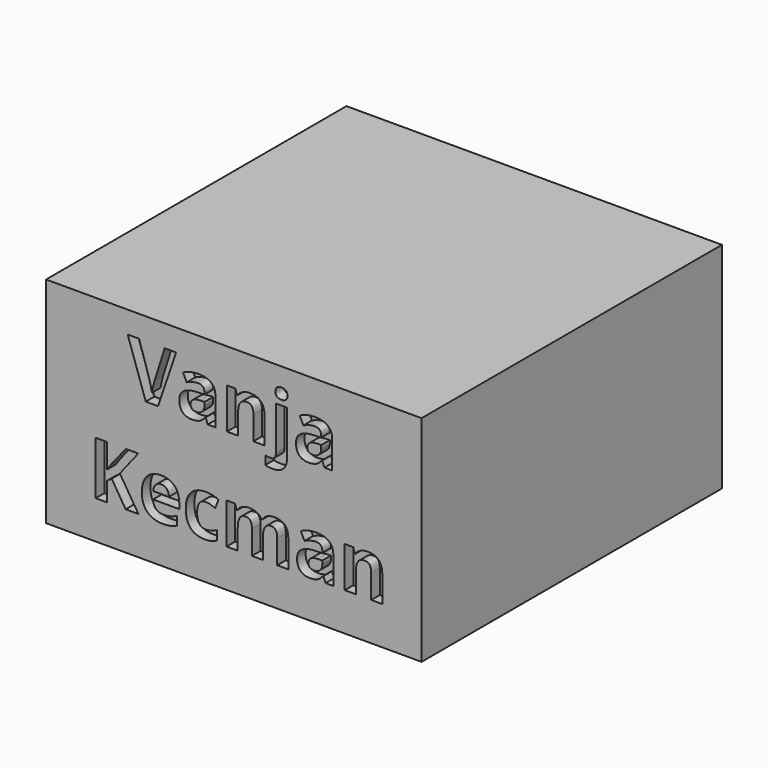
from build123d import *

# Parameters (mm, degrees)
F0_W         = 35
F0_H         = 35
F1_DEPTH     = 20
F2_TEXT_SIZE = 6.9444444444
F3_DEPTH     = 1


# Not quite as in the source:
# - Text() gives the source's letters only with a copy of the font that has no kerning and outlines rounded to 1/6400 em; it was checked with that copy


with BuildPart() as f1:
    # F0 (on Top) → F1 (new body)
    with BuildSketch(Plane.XY):
        with Locations((17.5, 17.5)):
            Rectangle(F0_W, F0_H)
    extrude(amount=F1_DEPTH)

    # F2 (on face) → F3 (cut)
    with BuildSketch(Plane.XZ):
        with Locations((7.6089409722, 13)):
            Text('Vanja', F2_TEXT_SIZE, font='Open Sans', font_style=FontStyle.BOLD, text_align=(TextAlign.LEFT, TextAlign.BOTTOM))
        with Locations((4, 3.5555555556)):
            Text('Kecman', F2_TEXT_SIZE, font='Open Sans', font_style=FontStyle.BOLD, text_align=(TextAlign.LEFT, TextAlign.BOTTOM))
    extrude(amount=-F3_DEPTH, mode=Mode.SUBTRACT)


solid = f1.part
